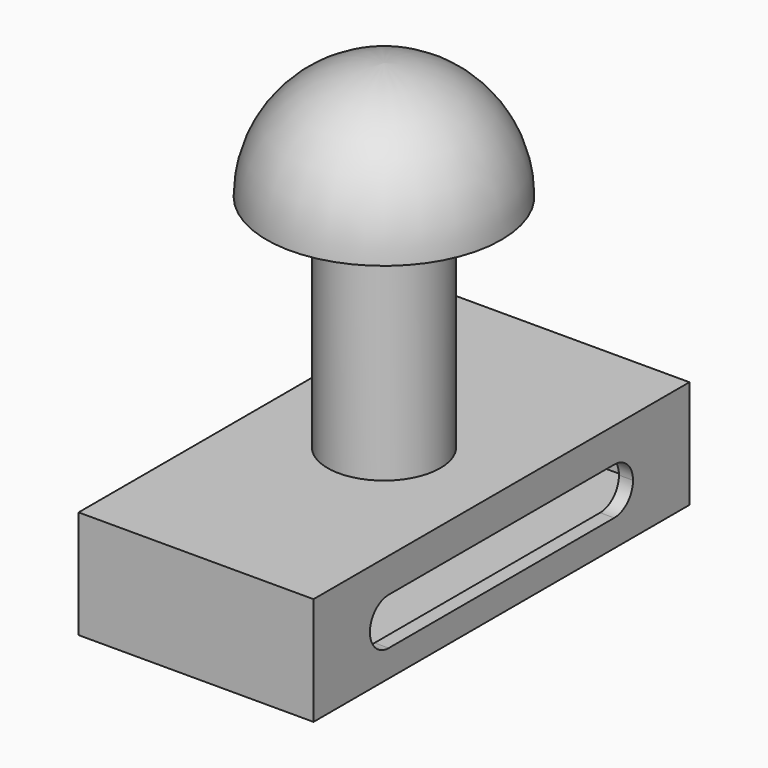
from build123d import *

# Parameters (mm, degrees)
F0_W      = 50
F0_H      = 100
F0_W_2    = 44
F0_H_2    = 94
F1_DEPTH  = 20
F2_DEPTH  = 3
F3_R      = 12
F4_DEPTH  = 3
F5_DEPTH  = 50
F6_R      = 25
F6_R_2    = 12
F7_DEPTH  = 25
F8_R      = 24.99999
F10_DEPTH = 30


# Not quite as in the source:
# - a fillet or chamfer is up to 0.001 mm smaller than in the source, because OpenCascade refuses the exact size
# - a feature names something its author has since deleted; it is built from what else it names


with BuildPart() as f1:
    # F0 (on Top) → F1 (new body)
    with BuildSketch(Plane.XY):
        Rectangle(F0_W, F0_H)
        Rectangle(F0_W_2, F0_H_2, mode=Mode.SUBTRACT)
    extrude(amount=F1_DEPTH)

    # F0 (on Top) → F2 (join)
    with BuildSketch(Plane.XY):
        Rectangle(F0_W, F0_H)
        Rectangle(F0_W_2, F0_H_2, mode=Mode.SUBTRACT)
        Rectangle(F0_W_2, F0_H_2)
    extrude(amount=F2_DEPTH)

    # F3 (on face) → F4 (join)
    with BuildSketch(Plane.XY.offset(20)):
        with BuildLine():
            ThreePointArc((22, 11.874342087), (0, 25), (-22, 11.874342087))
            Line((-22, 11.874342087), (-22, -11.874342087))
            ThreePointArc((-22, -11.874342087), (0, -25), (22, -11.874342087))
            Line((22, -11.874342087), (22, 11.874342087))
        make_face()
        Circle(F3_R, mode=Mode.SUBTRACT)
        with BuildLine():
            ThreePointArc((22, -11.874342087), (0, -25), (-22, -11.874342087))
            Line((-22, -11.874342087), (-22, -47))
            Line((-22, -47), (22, -47))
            Line((22, -47), (22, -11.874342087))
        make_face()
        with BuildLine():
            Line((-22, 47), (-22, 11.874342087))
            ThreePointArc((-22, 11.874342087), (0, 25), (22, 11.874342087))
            Line((22, 11.874342087), (22, 47))
            Line((22, 47), (-22, 47))
        make_face()
        Circle(F3_R)
        with BuildLine():
            Line((25, 50), (-25, 50))
            Line((-25, 50), (-25, -5.13e-08))
            ThreePointArc((-25, -5.13e-08), (-24.2383992934, 6.1237243321), (-22, 11.874342087))
            Line((-22, 11.874342087), (-22, 47))
            Line((-22, 47), (22, 47))
            Line((22, 47), (22, 11.874342087))
            ThreePointArc((22, 11.874342087), (24.2383992871, 6.123724357), (25, 0))
            Line((25, 0), (25, 50))
        make_face()
        with BuildLine():
            ThreePointArc((-22, -11.874342087), (-24.2383992808, -6.1237243818), (-25, -5.13e-08))
            Line((-25, -5.13e-08), (-25, -50))
            Line((-25, -50), (25, -50))
            Line((25, -50), (25, 0))
            ThreePointArc((25, 0), (24.2383992871, -6.123724357), (22, -11.874342087))
            Line((22, -11.874342087), (22, -47))
            Line((22, -47), (-22, -47))
            Line((-22, -47), (-22, -11.874342087))
        make_face()
        with BuildLine():
            ThreePointArc((22, -11.874342087), (24.2383992871, -6.123724357), (25, 0))
            ThreePointArc((25, 0), (24.2383992871, 6.123724357), (22, 11.874342087))
            Line((22, 11.874342087), (22, -11.874342087))
        make_face()
        with BuildLine():
            ThreePointArc((-22, 11.874342087), (-24.2383992934, 6.1237243321), (-25, -5.13e-08))
            ThreePointArc((-25, -5.13e-08), (-24.2383992808, -6.1237243818), (-22, -11.874342087))
            Line((-22, -11.874342087), (-22, 11.874342087))
        make_face()
    extrude(amount=F4_DEPTH)

    # F3 (on face) → F5 (join)
    with BuildSketch(Plane.XY.offset(20)):
        Circle(F3_R)
    extrude(amount=F5_DEPTH)

    # F9 (on Right) → F10 (cut, symmetric)
    with BuildSketch(Plane.YZ):
        with BuildLine():
            ThreePointArc((-25, 10.7041401789), (-26.4644660941, 14.2396740848), (-30, 15.7041401789))
            ThreePointArc((-30, 15.7041401789), (-35, 10.7041401789), (-30, 5.7041401789))
            ThreePointArc((-30, 5.7041401789), (-26.4644660941, 7.1686062729), (-25, 10.7041401789))
        make_face()
        with BuildLine():
            ThreePointArc((30, 5.7041401789), (25, 10.7041401789), (30, 15.7041401789))
            Line((30, 15.7041401789), (-30, 15.7041401789))
            ThreePointArc((-30, 15.7041401789), (-26.4644660941, 14.2396740848), (-25, 10.7041401789))
            ThreePointArc((-25, 10.7041401789), (-26.4644660941, 7.1686062729), (-30, 5.7041401789))
            Line((-30, 5.7041401789), (30, 5.7041401789))
        make_face()
        with BuildLine():
            ThreePointArc((30, 5.7041401789), (33.5355339059, 7.1686062729), (35, 10.7041401789))
            ThreePointArc((35, 10.7041401789), (33.5355339059, 14.2396740848), (30, 15.7041401789))
            ThreePointArc((30, 15.7041401789), (25, 10.7041401789), (30, 5.7041401789))
        make_face()
    extrude(amount=F10_DEPTH, both=True, mode=Mode.SUBTRACT)


with BuildPart() as f7:
    # F6 (on face) → F7 (new body)
    with BuildSketch(Plane.XY.offset(70)):
        Circle(F6_R)
        Circle(F6_R_2, mode=Mode.SUBTRACT)
        Circle(F6_R_2)
    extrude(amount=F7_DEPTH)

    # F8 (radius 25 in the source; OpenCascade refuses exactly that, so slightly less here)
    f8_edges = [f7.edges().sort_by_distance(p)[0] for p in [
        (-25, 0, 95),
    ]]
    fillet(f8_edges, radius=F8_R)


solid = Compound([f1.part, f7.part])
